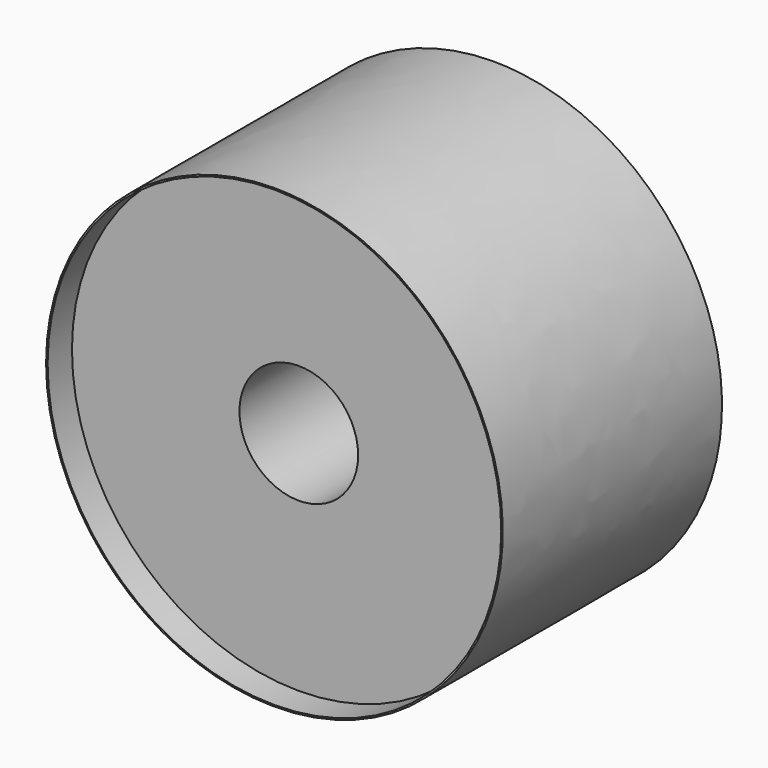
from build123d import *

# Parameters (mm, degrees)
F0_R     = 9.4610672483
F0_R_2   = 2.4756010363
F2_DEPTH = 10.16
F3_DEPTH = 11.43
F1_R     = 0.7289201881
F4_DEPTH = 12.319


with BuildPart() as f2:
    # F0 (on Front) → F2 (new body)
    with BuildSketch(Plane.XZ):
        Circle(F0_R)
        Circle(F0_R_2, mode=Mode.SUBTRACT)
    extrude(amount=F2_DEPTH)

    # F1 (on face) → F4 (cut)
    with BuildSketch(Plane.XZ):
        with Locations((-10.5307922242, 4.3296911371)):
            Circle(F1_R)
        with Locations((1.5157735968, -11.2847791566)):
            Circle(F1_R)
        with Locations((9.0150186273, 6.9550880195)):
            Circle(F1_R)
    extrude(amount=F4_DEPTH, mode=Mode.SUBTRACT)


with BuildPart() as f3:
    # F0 (on Front) → F3 (new body)
    with BuildSketch(Plane.XZ):
        with BuildLine():
            add(Edge.make_bspline(
                [(0, 9.525), (-16.4977839421, 9.525), (-8.248891971, -4.7625), (0, -19.05), (8.248891971, -4.7625), (16.4977839421, 9.525), (0, 9.525)],
                knots=[0, 0, 0, 2.0943951024, 2.0943951024, 4.1887902048, 4.1887902048, 6.2831853072, 6.2831853072, 6.2831853072], degree=2, weights=[1, 0.5, 1, 0.5, 1, 0.5, 1]))
        make_face()
        Circle(F0_R, mode=Mode.SUBTRACT)
    extrude(amount=F3_DEPTH)


solid = Compound([f2.part, f3.part])
